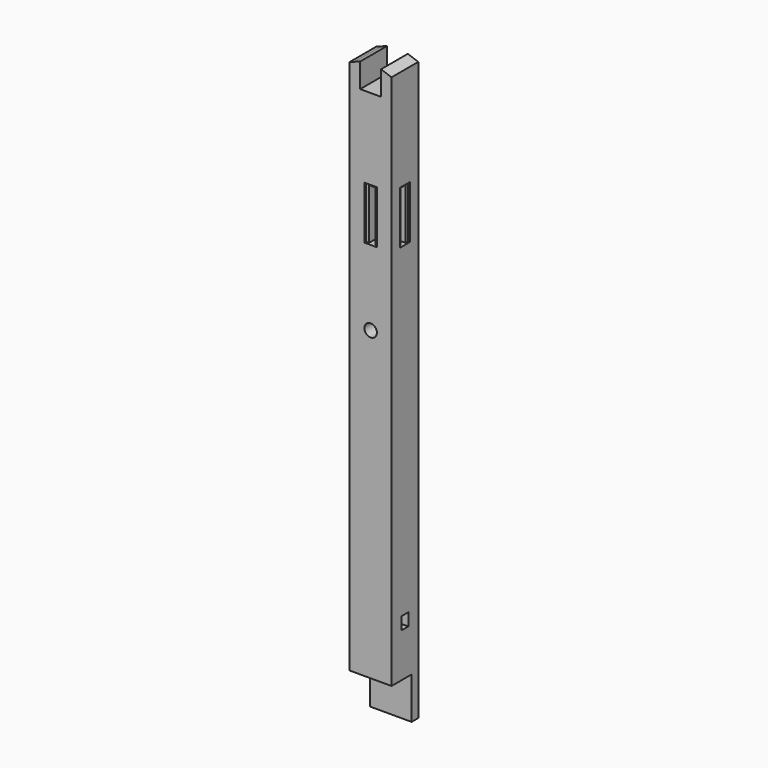
from build123d import *

# Parameters (mm, degrees)
F0_R      = 38.1
F0_W      = 38.1
F0_H      = 308.4068
F1_DEPTH  = 203.2
F2_DEPTH  = 76.2
F3_W      = 38.1
F3_H      = 308.4068
F4_DEPTH  = 76.2
F5_DEPTH  = 12.7
F6_DEPTH  = 12.7
F7_W      = 38.1
F7_H      = 308.4068
F8_DEPTH  = 76.2
F9_DEPTH  = 12.7
F10_W     = 38.1
F10_H     = 308.4068
F11_DEPTH = 76.2
F12_DEPTH = 12.7
F7_W_2    = 50.8
F7_H_2    = 76.2
F13_DEPTH = 254
F14_W     = 254
F14_H     = 50.8
F15_DEPTH = 254


# Not quite as in the source:
# - a feature names something its author has since deleted; it is built from what else it names


with BuildPart() as f1:
    # F0 (on Front) → F1 (new body)
    with BuildSketch(Plane.XZ):
        Polygon((-97.1309603494, 1586.2505768385), (-127, 1575.484752655), (-127, -1679.575), (127, -1679.575), (127, 1575.9600688261), (63.5, 1598.5777378082), (63.5, 1450.975), (-63.5, 1450.975), (-63.5, 1598.4984636307), (-97.1411935326, 1586.3062005624), align=None)
        with Locations((0, 180.975)):
            Circle(F0_R, mode=Mode.SUBTRACT)
        Polygon((19.05, 638.175), (-19.05, 638.175), (-38.1, 638.175), (-38.1, 959.2818), (38.1, 959.2818), (38.1, 638.175), align=None, mode=Mode.SUBTRACT)
        with Locations((0, 792.3784)):
            Rectangle(F0_W, F0_H)
        Polygon((-19.05, 638.175), (-19.05, 946.5818), (19.05, 946.5818), (19.05, 638.175), (38.1, 638.175), (38.1, 959.2818), (-38.1, 959.2818), (-38.1, 638.175), align=None)
    extrude(amount=F1_DEPTH)

    # F0 (on Front) → F2 (cut)
    with BuildSketch(Plane.XZ):
        with Locations((0, 792.3784)):
            Rectangle(F0_W, F0_H)
    extrude(amount=F2_DEPTH, mode=Mode.SUBTRACT)

    # F3 (on face) → F4 (cut)
    with BuildSketch(Plane.XZ.offset(203.2)):
        with Locations((0, 792.3784)):
            Rectangle(F3_W, F3_H)
    extrude(amount=-F4_DEPTH, mode=Mode.SUBTRACT)

    # F3 (on face) → F5 (cut)
    with BuildSketch(Plane.XZ.offset(203.2)):
        Polygon((-38.1, 638.175), (-19.05, 638.175), (-19.05, 946.5818), (19.05, 946.5818), (19.05, 638.175), (38.1, 638.175), (38.1, 959.2818), (-38.1, 959.2818), align=None)
    extrude(amount=-F5_DEPTH, mode=Mode.SUBTRACT)

    # F0 (on Front) → F6 (cut)
    with BuildSketch(Plane.XZ):
        Polygon((-19.05, 638.175), (-19.05, 946.5818), (19.05, 946.5818), (19.05, 638.175), (38.1, 638.175), (38.1, 959.2818), (-38.1, 959.2818), (-38.1, 638.175), align=None)
    extrude(amount=F6_DEPTH, mode=Mode.SUBTRACT)

    # F7 (on face) → F8 (cut)
    with BuildSketch(Plane.YZ.offset(127)):
        with Locations((-101.6, 792.3784)):
            Rectangle(F7_W, F7_H)
    extrude(amount=-F8_DEPTH, mode=Mode.SUBTRACT)

    # F7 (on face) → F9 (cut)
    with BuildSketch(Plane.YZ.offset(127)):
        Polygon((-139.7, 638.175), (-120.65, 638.175), (-120.65, 946.5818), (-82.55, 946.5818), (-82.55, 638.175), (-63.5, 638.175), (-63.5, 959.2818), (-139.7, 959.2818), align=None)
    extrude(amount=-F9_DEPTH, mode=Mode.SUBTRACT)

    # F10 (on face) → F11 (cut)
    with BuildSketch(Plane(origin=(-127, 0, 0), x_dir=(0, -1, 0), z_dir=(-1, 0, 0))):
        with Locations((101.6, 792.3784)):
            Rectangle(F10_W, F10_H)
    extrude(amount=-F11_DEPTH, mode=Mode.SUBTRACT)

    # F10 (on face) → F12 (cut)
    with BuildSketch(Plane(origin=(-127, 0, 0), x_dir=(0, -1, 0), z_dir=(-1, 0, 0))):
        Polygon((63.5, 638.175), (82.55, 638.175), (82.55, 946.5818), (120.65, 946.5818), (120.65, 638.175), (139.7, 638.175), (139.7, 959.2818), (63.5, 959.2818), align=None)
    extrude(amount=-F12_DEPTH, mode=Mode.SUBTRACT)

    # F7 (on face) → F13 (cut)
    with BuildSketch(Plane.YZ.offset(127)):
        with Locations((-100.9582259417, -1374.775)):
            Rectangle(F7_W_2, F7_H_2)
    extrude(amount=-F13_DEPTH, mode=Mode.SUBTRACT)

    # F14 (on face) → F15 (join)
    with BuildSketch(Plane(origin=(0, 0, -1679.575), x_dir=(1, 0, 0), z_dir=(0, 0, -1))):
        with Locations((0, 25.4)):
            Rectangle(F14_W, F14_H)
    extrude(amount=F15_DEPTH)


solid = f1.part
